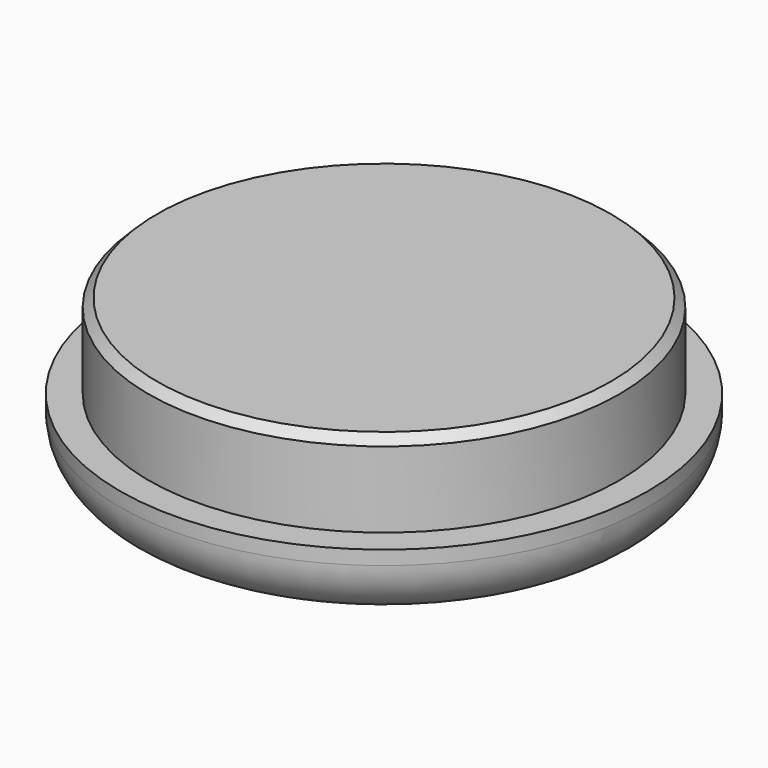
from build123d import *

# Parameters (mm, degrees)
F0_R         = 23.876
F1_DEPTH     = 6.35
F2_R         = 21.2725
F3_DEPTH     = 7.62
F4_R         = 5.08
F5_TEXT_SIZE = 12.6039699858
F6_DEPTH     = 0.635
F7_SIZE      = 0.762


# Not quite as in the source:
# - Text() gives the source's letters only with a copy of the font that has no kerning and outlines rounded to 1/6400 em; it was checked with that copy


with BuildPart() as f1:
    # F0 (on Top) → F1 (new body)
    with BuildSketch(Plane.XY):
        Circle(F0_R)
    extrude(amount=F1_DEPTH)

    # F2 (on face) → F3 (join)
    with BuildSketch(Plane.XY.offset(6.35)):
        Circle(F2_R)
    extrude(amount=F3_DEPTH)

    # F4
    f4_edges = [f1.edges().sort_by_distance(p)[0] for p in [
        (-23.876, 0, 0),
    ]]
    fillet(f4_edges, radius=F4_R)

    # F5 (on face) → F6 (cut)
    with BuildSketch(Plane(origin=(0, 0, 0), x_dir=(1, 0, 0), z_dir=(0, 0, -1))):
        with Locations((-7.2431607405, -5.0981203385)):
            Text('SD', F5_TEXT_SIZE, font='Open Sans', font_style=FontStyle.BOLD, text_align=(TextAlign.LEFT, TextAlign.BOTTOM))
    extrude(amount=-F6_DEPTH, mode=Mode.SUBTRACT)

    # F7
    f7_edges = [f1.edges().sort_by_distance(p)[0] for p in [
        (-21.2725, 0, 13.97),
    ]]
    chamfer(f7_edges, length=F7_SIZE)


solid = f1.part
